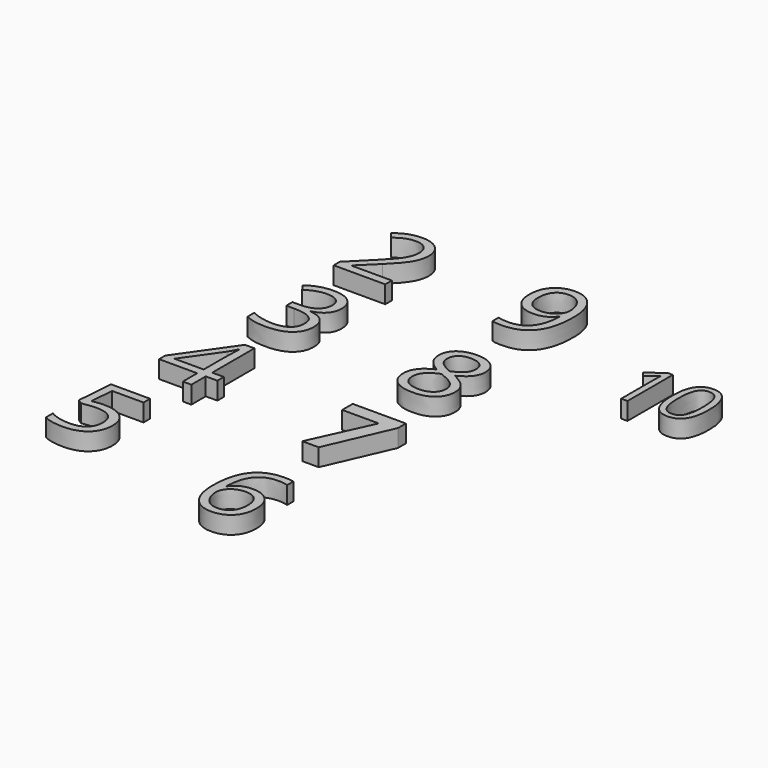
from build123d import *

# Parameters (mm, degrees)
F0_TEXT_SIZE   = 12.5
F0_TEXT_SIZE_2 = 11.8055555556
F0_TEXT_SIZE_3 = 9.0277777778
F1_DEPTH       = 2


# Not quite as in the source:
# - a feature names something its author has since deleted; it is built from what else it names
# - Text() gives the source's letters only with a copy of the font that has no kerning and outlines rounded to 1/6400 em; it was checked with that copy


with BuildPart() as f1:
    # F0 (on Top) → F1 (new body)
    with BuildSketch(Plane.XY):
        with Locations((-59.0959224531, 54.3187791963)):
            Text('2', F0_TEXT_SIZE, font='Open Sans', text_align=(TextAlign.LEFT, TextAlign.BOTTOM))
        with Locations((-58.8613385947, 41.4486846903)):
            Text('3', F0_TEXT_SIZE, font='Open Sans', text_align=(TextAlign.LEFT, TextAlign.BOTTOM))
        with Locations((-59.5804257931, 28.4661651139)):
            Text('4', F0_TEXT_SIZE, font='Open Sans', text_align=(TextAlign.LEFT, TextAlign.BOTTOM))
        with Locations((-42.0532362607, 54.7542874401)):
            Text('9', F0_TEXT_SIZE, font='Open Sans', text_align=(TextAlign.LEFT, TextAlign.BOTTOM))
        with Locations((-41.30912759, 39.7222605233)):
            Text('8', F0_TEXT_SIZE, font='Open Sans', text_align=(TextAlign.LEFT, TextAlign.BOTTOM))
        with Locations((-40.8205632733, 26.132010821)):
            Text('7', F0_TEXT_SIZE_2, font='Open Sans', font_style=FontStyle.BOLD, text_align=(TextAlign.LEFT, TextAlign.BOTTOM))
        with Locations((-60.9832811782, 15.1440059317)):
            Text('5', F0_TEXT_SIZE, font='Open Sans', text_align=(TextAlign.LEFT, TextAlign.BOTTOM))
        with Locations((-41.1358834857, 10.637836579)):
            Text('6', F0_TEXT_SIZE, font='Open Sans', text_align=(TextAlign.LEFT, TextAlign.BOTTOM))
        with Locations((-24.9294252748, 50.2338564133)):
            Text('10', F0_TEXT_SIZE_3, font='Open Sans', text_align=(TextAlign.LEFT, TextAlign.BOTTOM))
    extrude(amount=F1_DEPTH)


solid = f1.part
